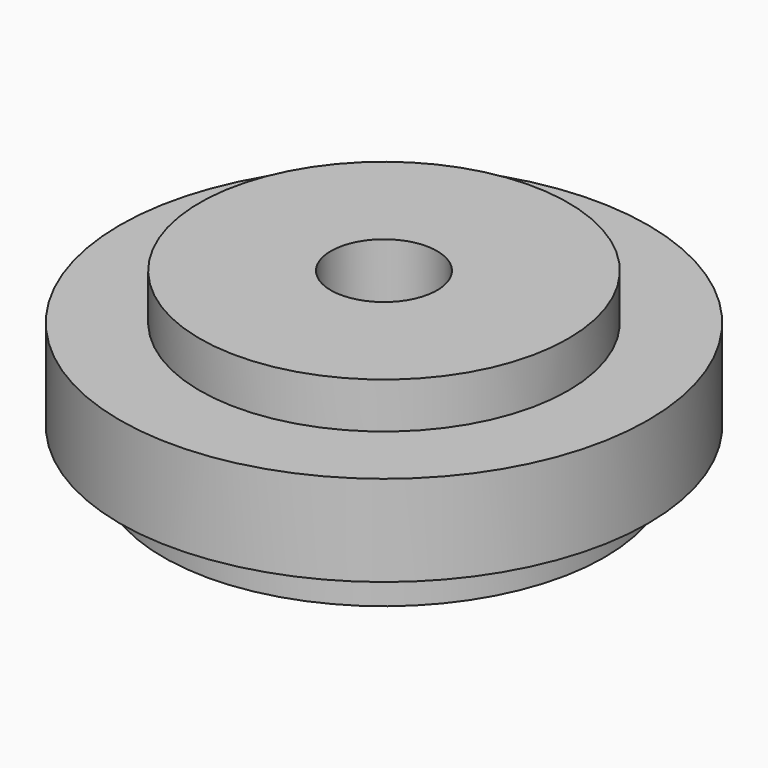
from build123d import *

# Parameters (mm, degrees)
F0_R     = 10.4775
F1_DEPTH = 10.2743
F0_R_2   = 12.5476
F2_DEPTH = 7.6708
F3_START = 2.5019
F0_R_3   = 15.0241
F3_DEPTH = 5.1689
F4_D     = 6.0452


# Not quite as in the source:
# - a feature names something its author has since deleted; it is built from what else it names


with BuildPart() as f1:
    # F0 (on Top) → F1 (new body)
    with BuildSketch(Plane.XY):
        Circle(F0_R)
    extrude(amount=F1_DEPTH)

    # F0 (on Top) → F2 (join)
    with BuildSketch(Plane.XY):
        Circle(F0_R_2)
        Circle(F0_R, mode=Mode.SUBTRACT)
    extrude(amount=F2_DEPTH)

    # F0 (on Top) → F3 (join)
    with BuildSketch(Plane.XY.offset(F3_START)):
        Circle(F0_R_3)
        Circle(F0_R_2, mode=Mode.SUBTRACT)
    extrude(amount=F3_DEPTH)

    # F4 (through all)
    with Locations(Plane(origin=(0, 0, 0), x_dir=(1, 0, 0), z_dir=(0, 0, -1))):
        with Locations((0, 0)):
            Hole(F4_D / 2)


solid = f1.part
